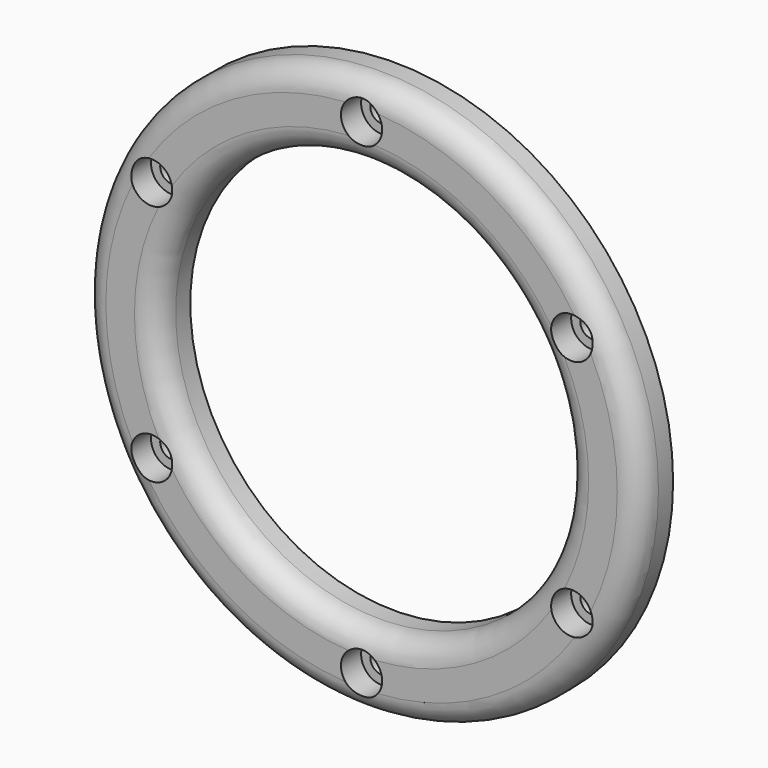
from build123d import *

# Parameters (mm, degrees)
F0_R     = 30.9245
F0_R_2   = 22.6695
F1_DEPTH = 4.572
F2_R     = 29.5275
F2_R_2   = 24.3205
F3_DEPTH = 1.905
F4_R     = 3.81
F5_DEPTH = 0.889
F6_R     = 1.27
F7_DEPTH = 3.557
F8_R     = 2.286
F9_DEPTH = 2.794


# Not quite as in the source:
# - a fillet or chamfer that OpenCascade refuses, or shapes differently, is made with other operations: its cross-section is extruded or revolved along the edge and cut away or added


with BuildPart() as f1:
    # F0 (on Front) → F1 (new body)
    with BuildSketch(Plane.XZ):
        Circle(F0_R)
        Circle(F0_R_2, mode=Mode.SUBTRACT)
    extrude(amount=F1_DEPTH)

    # F2 (on face) → F3 (cut)
    with BuildSketch(Plane(origin=(0, 0, 0), x_dir=(-1, 0, 0), z_dir=(0, 1, 0))):
        Circle(F2_R)
        Circle(F2_R_2, mode=Mode.SUBTRACT)
    extrude(amount=-F3_DEPTH, mode=Mode.SUBTRACT)

    # F4 (on face) → F5 (join)
    with BuildSketch(Plane(origin=(0, -1.905, 0), x_dir=(-1, 0, 0), z_dir=(0, 1, 0))):
        with Locations((0, 26.924)):
            Circle(F4_R)
        with Locations((-23.3168679715, 13.462)):
            Circle(F4_R)
        with Locations((-23.3168679715, -13.462)):
            Circle(F4_R)
        with Locations((0, -26.924)):
            Circle(F4_R)
        with Locations((23.3168679715, -13.462)):
            Circle(F4_R)
        with Locations((23.3168679715, 13.462)):
            Circle(F4_R)
    extrude(amount=F5_DEPTH)

    # F6 (on face) → F7 (cut, through all)
    with BuildSketch(Plane(origin=(0, -1.016, 0), x_dir=(-1, 0, 0), z_dir=(0, 1, 0))):
        with Locations((0, 26.924)):
            Circle(F6_R)
        with Locations((-23.3168679715, 13.462)):
            Circle(F6_R)
        with Locations((-23.3168679715, -13.462)):
            Circle(F6_R)
        with Locations((0, -26.924)):
            Circle(F6_R)
        with Locations((23.3168679715, -13.462)):
            Circle(F6_R)
        with Locations((23.3168679715, 13.462)):
            Circle(F6_R)
    extrude(amount=-F7_DEPTH, mode=Mode.SUBTRACT)

    # F8 (on face) → F9 (cut)
    with BuildSketch(Plane.XZ.offset(4.572)):
        with Locations((0, 26.924)):
            Circle(F8_R)
        with Locations((-23.3168679715, 13.462)):
            Circle(F8_R)
        with Locations((-23.3168679715, -13.462)):
            Circle(F8_R)
        with Locations((0, -26.924)):
            Circle(F8_R)
        with Locations((23.3168679715, -13.462)):
            Circle(F8_R)
        with Locations((23.3168679715, 13.462)):
            Circle(F8_R)
    extrude(amount=-F9_DEPTH, mode=Mode.SUBTRACT)

    # F10: fillet of radius 2.54 on 2 edges, made by hand

    # F10_s1 → F10_t2 (revolve, cut)
    with BuildSketch(Plane.XY):
        with BuildLine():
            ThreePointArc((30.9245, -2.032), (30.1805512242, -3.8280512242), (28.3845, -4.572))
            Line((28.3845, -4.572), (30.9245, -4.572))
            Line((30.9245, -4.572), (30.9245, -2.032))
        make_face()
    revolve(axis=Axis((0, -4.572, 0), (0, -1, 0)), mode=Mode.SUBTRACT)

    # F10_s3 → F10_t4 (revolve, cut)
    with BuildSketch(Plane.XY):
        with BuildLine():
            ThreePointArc((25.2095, -4.572), (23.4134487758, -3.8280512242), (22.6695, -2.032))
            Line((22.6695, -2.032), (22.6695, -4.572))
            Line((22.6695, -4.572), (25.2095, -4.572))
        make_face()
    revolve(axis=Axis((0, -4.572, 0), (0, -1, 0)), mode=Mode.SUBTRACT)


solid = f1.part
